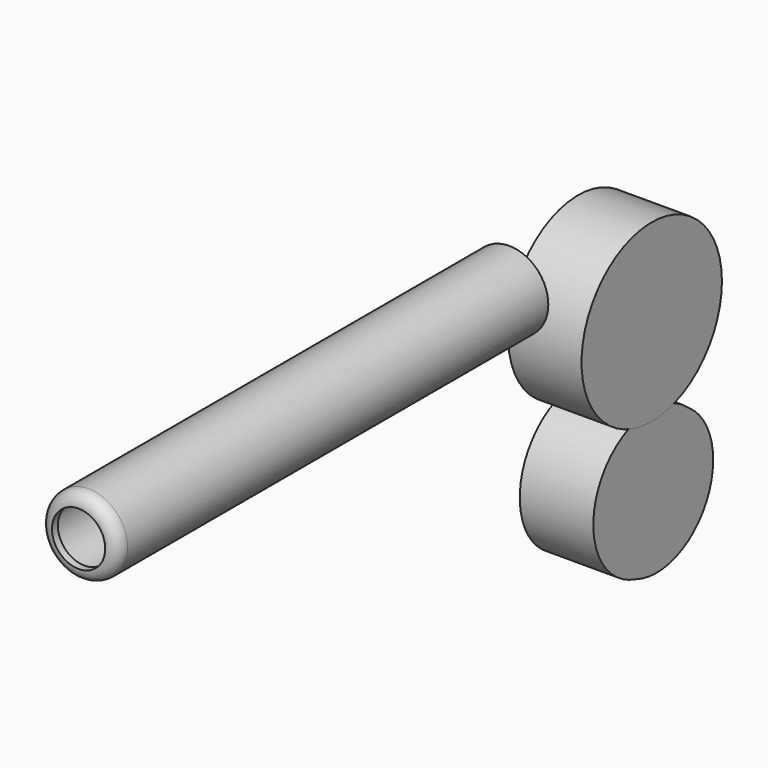
from build123d import *

# Parameters (mm, degrees)
F0_R      = 13.4869119151
F1_DEPTH  = 185.928
F2_R      = 4.2924717139
F3_T      = -2.54
F4_R      = 24.8992678704
F5_DEPTH  = 25.4
F6_R      = 24.4404976371
F5_FACE_R = 24.8992678704
F7_DEPTH  = 25.4
F8_R      = 30.2953984927
F9_DEPTH  = 25.4


# Not quite as in the source:
# - a shell that OpenCascade refuses in one call is made with other operations: the cavity is built on its own and cut out


with BuildPart() as f1:
    # F0 (on Front) → F1 (new body)
    with BuildSketch(Plane.XZ):
        Circle(F0_R)
    extrude(amount=F1_DEPTH)

    # F2
    f2_edges = [f1.edges().sort_by_distance(p)[0] for p in [
        (-13.486912, -185.928, 0),
    ]]
    fillet(f2_edges, radius=F2_R)

    # F3: a shell. OpenCascade refuses it in one call, so the cavity is built on its own and cut out:
    # the body offset inwards by the wall thickness, plus a prism from it out through each open face.
    f3_core = offset(f1.part, amount=F3_T, mode=Mode.PRIVATE)
    f3_exits = [f3_core.faces().sort_by_distance(p)[0] for p in [
        (0, -183.388, 0),
    ]]
    add(f3_core, mode=Mode.SUBTRACT)
    extrude(f3_exits, amount=-F3_T, mode=Mode.SUBTRACT)


with BuildPart() as f5:
    # F4 (on Right) → F5 (new body)
    with BuildSketch(Plane.YZ):
        with Locations((29.4352918863, -64.9161785841)):
            Circle(F4_R)
    extrude(amount=F5_DEPTH)

    # F6 (on Right) + F5_face (on face) → F7 (join)
    with BuildSketch(Plane.YZ):
        with Locations((31.84100613, -66.205278039)):
            Circle(F6_R)
    with BuildSketch(Plane(origin=(0, 29.4352918863, -64.9161785841), x_dir=(0, 1, 0), z_dir=(-1, 0, 0))):
        Circle(F5_FACE_R)
    extrude(amount=F7_DEPTH, dir=(1, 0, 0))


with BuildPart() as f9:
    # F8 (on Right) → F9 (new body)
    with BuildSketch(Plane.YZ):
        with Locations((29.7687537968, -13.4697174653)):
            Circle(F8_R)
    extrude(amount=F9_DEPTH)


solid = Compound([f1.part, f5.part, f9.part])
